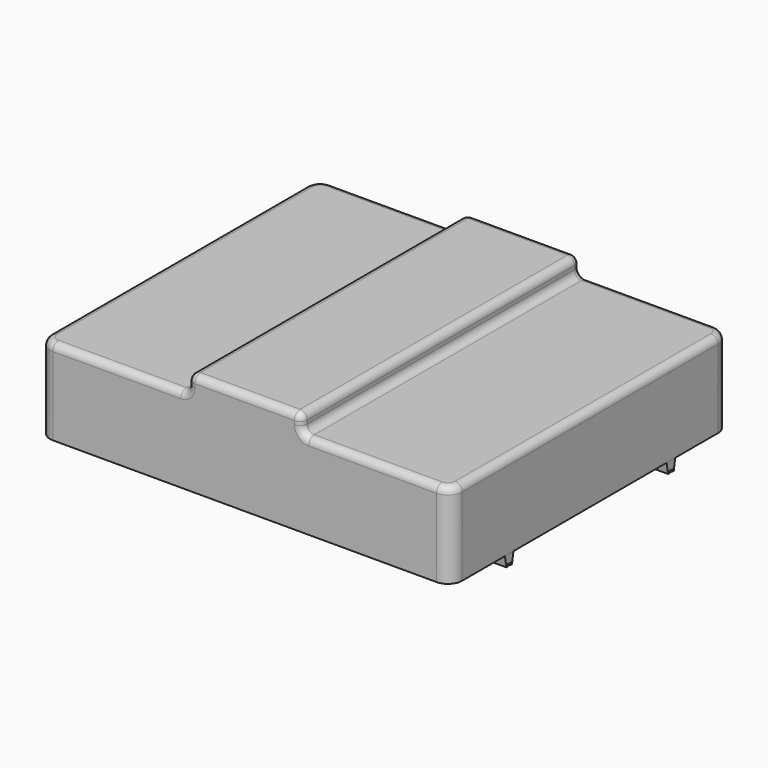
from build123d import *

# Parameters (mm, degrees)
F0_W         = 1473.2
F0_H         = 1244.6
F1_DEPTH     = 304.8
F2_W         = 406.4
F2_H         = 1244.6
F3_DEPTH     = 63.5
F5_F1_R      = 25.4
F5_F2_R      = 25.4
F6_T1_DEPTH  = 431.8
F6_T4_ANGLE  = 90
F6_T6_ANGLE  = 90
F6_T8_ANGLE  = 90
F6_T10_ANGLE = 90
F8_DEPTH     = 1473.2


# Not quite as in the source:
# - a fillet or chamfer that OpenCascade refuses, or shapes differently, is made with other operations: its cross-section is extruded or revolved along the edge and cut away or added
# - a feature of the source that left no trace in its solid (it failed there, or was rolled back) is left out


with BuildPart() as f1:
    # F0 (on Top) → F1 (new body)
    with BuildSketch(Plane.XY):
        Rectangle(F0_W, F0_H)
    extrude(amount=F1_DEPTH)

    # F2 (on face) → F3 (join)
    with BuildSketch(Plane.XY.offset(304.8)):
        Rectangle(F2_W, F2_H)
    extrude(amount=F3_DEPTH)

    # F5: fillet of radius 25.4 on 12 edges, made by hand

    # F5_f1
    f5_f1_edges = [f1.edges().sort_by_distance(p)[0] for p in [
        (-203.2, 0, 304.8),
        (203.2, 0, 304.8),
    ]]
    fillet(f5_f1_edges, radius=F5_F1_R)

    # F5_f2
    f5_f2_edges = [f1.edges().sort_by_distance(p)[0] for p in [
        (-482.6, -622.3, 304.8),
        (482.6, -622.3, 304.8),
        (736.6, 0, 304.8),
        (482.6, 622.3, 304.8),
        (-482.6, 622.3, 304.8),
        (-736.6, 0, 304.8),
        (0, 622.3, 368.3),
        (0, -622.3, 368.3),
        (-203.2, 0, 368.3),
        (203.2, 0, 368.3),
        (-210.6394877579, 622.3, 312.2394877579),
        (210.6394877579, 622.3, 312.2394877579),
        (210.6394877579, -622.3, 312.2394877579),
        (-210.6394877579, -622.3, 312.2394877579),
    ]]
    fillet(f5_f2_edges, radius=F5_F2_R)

    # F6: fillet of radius 50.8 on 4 edges, made by hand

    # F6_s2 → F6_t1 (cut)
    with BuildSketch(Plane.XY.offset(-127)):
        with BuildLine():
            ThreePointArc((736.6, -571.5), (721.7210244843, -607.4210244843), (685.8, -622.3))
            Line((685.8, -622.3), (736.6, -622.3))
            Line((736.6, -622.3), (736.6, -571.5))
        make_face()
        with BuildLine():
            ThreePointArc((685.8, 622.3), (721.7210244843, 607.4210244843), (736.6, 571.5))
            Line((736.6, 571.5), (736.6, 622.3))
            Line((736.6, 622.3), (685.8, 622.3))
        make_face()
        with BuildLine():
            ThreePointArc((-685.8, 622.3), (-721.7210244843, 607.4210244843), (-736.6, 571.5))
            Line((-736.6, 571.5), (-736.6, 622.3))
            Line((-736.6, 622.3), (-685.8, 622.3))
        make_face()
        with BuildLine():
            ThreePointArc((-736.6, -571.5), (-721.7210244843, -607.4210244843), (-685.8, -622.3))
            Line((-685.8, -622.3), (-736.6, -622.3))
            Line((-736.6, -622.3), (-736.6, -571.5))
        make_face()
    extrude(amount=F6_T1_DEPTH, mode=Mode.SUBTRACT)

    # F6_s3 → F6_t4 (revolve, cut)
    with BuildSketch(Plane.XZ.offset(571.5)):
        with BuildLine():
            ThreePointArc((-711.2, 304.8), (-729.1605122421, 297.3605122421), (-736.6, 279.4))
            Line((-736.6, 279.4), (-736.6, 304.8))
            Line((-736.6, 304.8), (-711.2, 304.8))
        make_face()
    revolve(axis=Axis((-685.8, -571.5, 304.8), (0, 0, 1)), revolution_arc=F6_T4_ANGLE, mode=Mode.SUBTRACT)

    # F6_s5 → F6_t6 (revolve, cut)
    with BuildSketch(Plane.YZ.offset(-685.8)):
        with BuildLine():
            ThreePointArc((596.9, 304.8), (614.8605122421, 297.3605122421), (622.3, 279.4))
            Line((622.3, 279.4), (622.3, 304.8))
            Line((622.3, 304.8), (596.9, 304.8))
        make_face()
    revolve(axis=Axis((-685.8, 571.5, 304.8), (0, 0, 1)), revolution_arc=F6_T6_ANGLE, mode=Mode.SUBTRACT)

    # F6_s7 → F6_t8 (revolve, cut)
    with BuildSketch(Plane.XZ.offset(-571.5)):
        with BuildLine():
            ThreePointArc((711.2, 304.8), (729.1605122421, 297.3605122421), (736.6, 279.4))
            Line((736.6, 279.4), (736.6, 304.8))
            Line((736.6, 304.8), (711.2, 304.8))
        make_face()
    revolve(axis=Axis((685.8, 571.5, 304.8), (0, 0, 1)), revolution_arc=F6_T8_ANGLE, mode=Mode.SUBTRACT)

    # F6_s9 → F6_t10 (revolve, cut)
    with BuildSketch(Plane.YZ.offset(685.8)):
        with BuildLine():
            ThreePointArc((-596.9, 304.8), (-614.8605122421, 297.3605122421), (-622.3, 279.4))
            Line((-622.3, 279.4), (-622.3, 304.8))
            Line((-622.3, 304.8), (-596.9, 304.8))
        make_face()
    revolve(axis=Axis((685.8, -571.5, 304.8), (0, 0, 1)), revolution_arc=F6_T10_ANGLE, mode=Mode.SUBTRACT)


with BuildPart() as f8:
    # F7 (on face) → F8 (new body)
    with BuildSketch(Plane.YZ.offset(736.6)):
        Polygon((-342.3026821136, 0), (-361.3526821136, 0), (-380.4026821136, 0), (-374.042391777, -38.1048284471), (-365.658134222, -38.1048284471), (-365.658134222, -34.2525914311), (-370.6433773041, -34.2525914311), (-370.6433773041, -30.6269582361), (-361.3526821136, -30.6269582361), (-352.0619869232, -30.6269582361), (-352.0619869232, -34.2525914311), (-357.0472300053, -34.2525914311), (-357.0472300053, -38.1048284471), (-348.6629724503, -38.1048284471), align=None)
    extrude(amount=-F8_DEPTH)


with BuildPart() as f8b:
    # F7 (on face) → F8, piece 2 (new body)
    with BuildSketch(Plane.YZ.offset(736.6)):
        Polygon((361.3526821136, 0), (342.3026821136, 0), (348.6629724503, -38.1048284471), (357.0472300053, -38.1048284471), (357.0472300053, -34.2525914311), (352.0619869232, -34.2525914311), (352.0619869232, -30.6269582361), (361.3526821136, -30.6269582361), (370.6433773041, -30.6269582361), (370.6433773041, -34.2525914311), (365.658134222, -34.2525914311), (365.658134222, -38.1048284471), (374.042391777, -38.1048284471), (380.4026821136, 0), align=None)
    extrude(amount=-F8_DEPTH)


solid = Compound([f1.part, f8.part, f8b.part])
